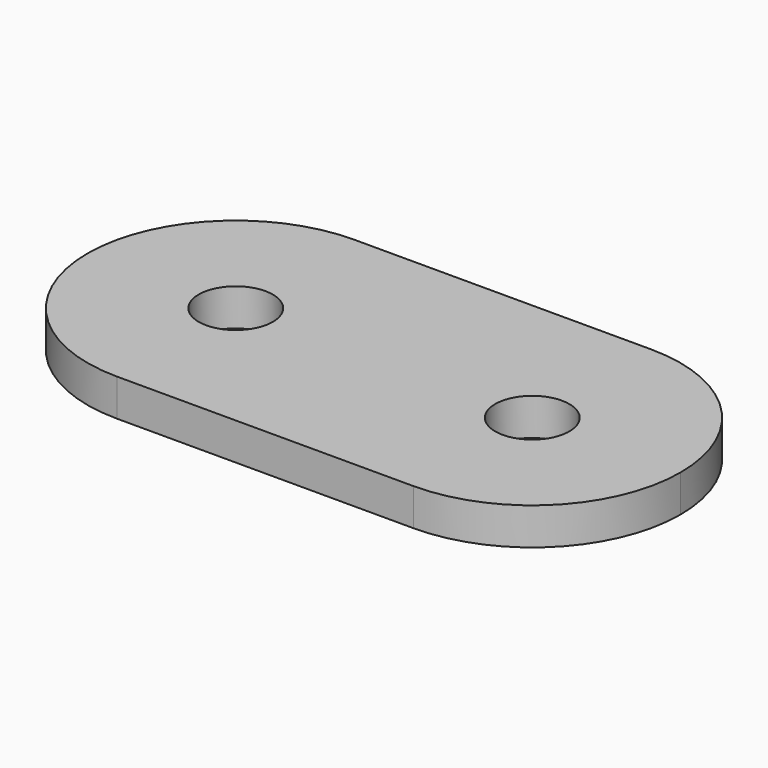
from build123d import *

# Parameters (mm, degrees)
F0_W     = 101.6
F0_H     = 50.8
F1_DEPTH = 3.175
F2_R     = 25.39999
F4_D     = 12.7


# Not quite as in the source:
# - a fillet or chamfer is up to 0.001 mm smaller than in the source, because OpenCascade refuses the exact size


with BuildPart() as f1:
    # F0 (on Top) → F1 (new body, symmetric)
    with BuildSketch(Plane.XY):
        Rectangle(F0_W, F0_H)
    extrude(amount=F1_DEPTH, both=True)

    # F2 (radius 25.4 in the source; OpenCascade refuses exactly that, so slightly less here)
    f2_edges = [f1.edges().sort_by_distance(p)[0] for p in [
        (-50.8, -25.4, 0),
        (50.8, -25.4, 0),
        (50.8, 25.4, 0),
        (-50.8, 25.4, 0),
    ]]
    fillet(f2_edges, radius=F2_R)

    # F4 (through all)
    with Locations(Plane.XY.offset(3.175)):
        with Locations((25.4, 0), (-25.4, 0)):
            Hole(F4_D / 2)


solid = f1.part
